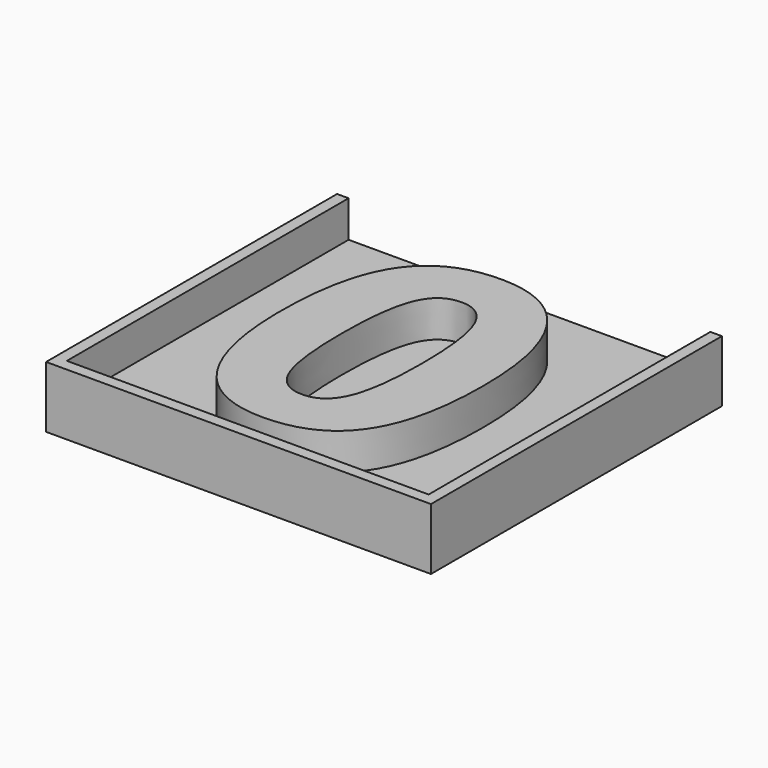
from build123d import *

# Parameters (mm, degrees)
F0_W         = 100
F0_H         = 91.5
F1_DEPTH     = 16
F2_W         = 94
F2_H         = 91.5
F3_DEPTH     = 9.5
F4_W         = 94
F4_H         = 28
F5_DEPTH     = 3.2
F6_TEXT_SIZE = 105.5555555556
F7_DEPTH     = 9.5
F8_W         = 100
F8_H         = 16
F9_DEPTH     = 3


# Not quite as in the source:
# - Text() gives the source's letters only with a copy of the font that has no kerning and outlines rounded to 1/6400 em; it was checked with that copy


with BuildPart() as f1:
    # F0 (on Top) → F1 (new body)
    with BuildSketch(Plane.XY):
        with Locations((50, 45.75)):
            Rectangle(F0_W, F0_H)
    extrude(amount=F1_DEPTH)

    # F2 (on face) → F3 (cut)
    with BuildSketch(Plane.XY.offset(16)):
        with Locations((50, 45.75)):
            Rectangle(F2_W, F2_H)
    extrude(amount=-F3_DEPTH, mode=Mode.SUBTRACT)

    # F4 (on face) → F5 (cut)
    with BuildSketch(Plane(origin=(0, 0, 0), x_dir=(1, 0, 0), z_dir=(0, 0, -1))):
        with Locations((50, -80.1)):
            Rectangle(F4_W, F4_H)
    extrude(amount=-F5_DEPTH, mode=Mode.SUBTRACT)

    # F6 (on face) → F7 (join)
    with BuildSketch(Plane.XY.offset(6.5)):
        with Locations((19.3666666667, 6.5)):
            Text('0', F6_TEXT_SIZE, font='Open Sans', font_style=FontStyle.BOLD, text_align=(TextAlign.LEFT, TextAlign.BOTTOM))
    extrude(amount=F7_DEPTH)

    # F8 (on face) → F9 (join)
    with BuildSketch(Plane.XZ):
        with Locations((50, 8)):
            Rectangle(F8_W, F8_H)
    extrude(amount=F9_DEPTH)


solid = f1.part
